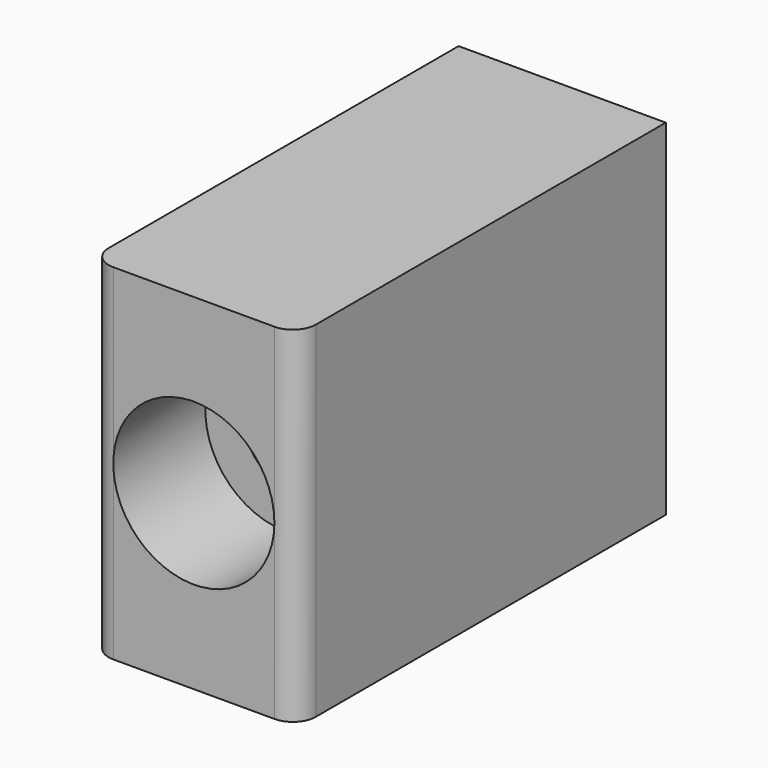
from build123d import *

# Parameters (mm, degrees)
F0_W     = 9
F0_H     = 15
F1_DEPTH = 20
F2_R     = 1.75
F3_DEPTH = 20.001
F4_R     = 3.5
F5_DEPTH = 5
F6_R     = 0.99999


# Not quite as in the source:
# - a fillet or chamfer is up to 0.001 mm smaller than in the source, because OpenCascade refuses the exact size


with BuildPart() as f1:
    # F0 (on Front) → F1 (new body)
    with BuildSketch(Plane.XZ):
        Rectangle(F0_W, F0_H)
    extrude(amount=F1_DEPTH)

    # F2 (on face) → F3 (cut, through all)
    with BuildSketch(Plane.XZ.offset(20)):
        Circle(F2_R)
    extrude(amount=-F3_DEPTH, mode=Mode.SUBTRACT)

    # F4 (on face) → F5 (cut)
    with BuildSketch(Plane.XZ.offset(20)):
        Circle(F4_R)
    extrude(amount=-F5_DEPTH, mode=Mode.SUBTRACT)

    # F6 (radius 1 in the source; OpenCascade refuses exactly that, so slightly less here)
    f6_edges = [f1.edges().sort_by_distance(p)[0] for p in [
        (4.5, -20, 0),
        (-4.5, -20, 0),
    ]]
    fillet(f6_edges, radius=F6_R)


solid = f1.part
